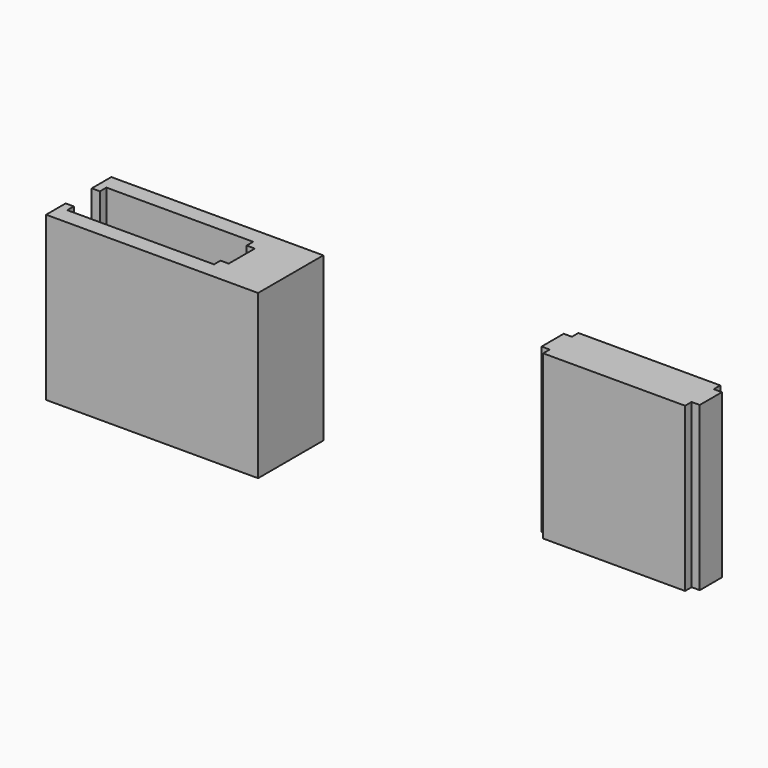
from build123d import *

# Parameters (mm, degrees)
F1_DEPTH = 25.4
F0_W     = 22.098
F0_H     = 4.318
F0_W_2   = 1.27
F0_H_2   = 1.27


# Not quite as in the source:
# - a feature names something its author has since deleted; it is built from what else it names


with BuildPart() as f1:
    # F0 (on Top) → F1 (new body)
    with BuildSketch(Plane.XY):
        Polygon((-20.1215016502, -3.8572545798), (-20.1215016502, -2.5872545798), (2.7384983498, -2.5872545798), (2.7384983498, -3.8572545798), (4.0084983498, -3.8572545798), (4.0084983498, -8.9372545798), (2.7384983498, -8.9372545798), (2.7384983498, -10.2072545798), (-20.1215016502, -10.2072545798), (-20.1215016502, -8.9372545798), (-21.3915016502, -8.9372545798), (-21.3915016502, -12.7472545798), (11.6284983498, -12.7472545798), (11.6284983498, -0.0472545798), (-21.3915016502, -0.0472545798), (-21.3915016502, -3.8572545798), align=None)
    extrude(amount=F1_DEPTH)


with BuildPart() as f1b:
    # F0 (on Top) → F1, piece 2 (new body)
    with BuildSketch(Plane.XY):
        with Locations((59.6792152276, -0.0636551082)):
            Rectangle(F0_W, F0_H)
        with Locations((47.9952152276, -0.0636551082)):
            Rectangle(F0_W_2, F0_H)
        with Locations((59.6792152276, -2.8576551082)):
            Rectangle(F0_W, F0_H_2)
        with Locations((59.6792152276, 2.7303448918)):
            Rectangle(F0_W, F0_H_2)
        with Locations((71.3632152276, -0.0636551082)):
            Rectangle(F0_W_2, F0_H)
    extrude(amount=F1_DEPTH)


solid = Compound([f1.part, f1b.part])
